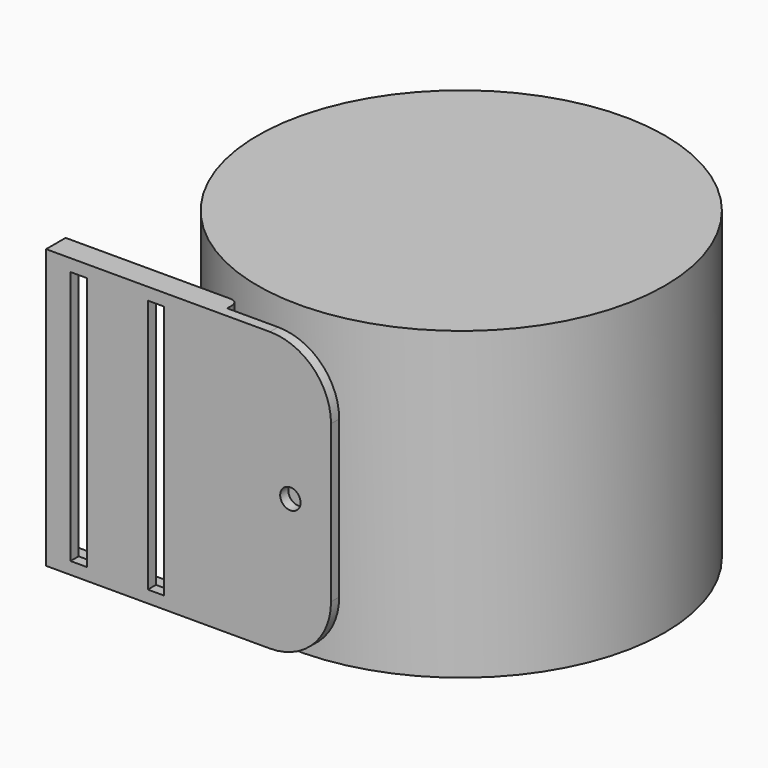
from build123d import *

# Parameters (mm, degrees)
F0_W        = 140
F0_H        = 137
F0_R        = 5
F0_W_2      = 8
F0_H_2      = 125
F1_DEPTH    = 5
F2_R        = 30
F3_R        = 30
F4_W        = 85
F4_H        = 7
F5_DEPTH    = 5
F6_T1_DEPTH = 132.5735082217
F7_W        = 85
F7_H        = 5
F8_DEPTH    = 7
F9_R        = 4
F10_R       = 100.0006041304
F11_DEPTH   = 150


# Not quite as in the source:
# - a fillet or chamfer that OpenCascade refuses, or shapes differently, is made with other operations: its cross-section is extruded or revolved along the edge and cut away or added


with BuildPart() as f1:
    # F0 (on Front) → F1 (new body)
    with BuildSketch(Plane.XZ):
        with Locations((-70, 68.5)):
            Rectangle(F0_W, F0_H)
        Polygon((-128, 5.9977934385), (-128, 130.9977934385), (-120, 130.9977934385), (-120, 6), (-120, 5.9977934385), align=None, mode=Mode.SUBTRACT)
        with Locations((-19.9747101513, 67.9977461696)):
            Circle(F0_R, mode=Mode.SUBTRACT)
        with Locations((-86, 68.5)):
            Rectangle(F0_W_2, F0_H_2, mode=Mode.SUBTRACT)
    extrude(amount=F1_DEPTH)

    # F2
    f2_edges = [f1.edges().sort_by_distance(p)[0] for p in [
        (0, -2.5, 137),
    ]]
    fillet(f2_edges, radius=F2_R)

    # F3
    f3_edges = [f1.edges().sort_by_distance(p)[0] for p in [
        (0, -2.5, 0),
    ]]
    fillet(f3_edges, radius=F3_R)

    # F4 (on Top) → F5 (join)
    with BuildSketch(Plane.XY):
        with Locations((-97.5, 3.5)):
            Rectangle(F4_W, F4_H)
    extrude(amount=F5_DEPTH)

    # F6: fillet of radius 50 on 1 edges, made by hand

    # F6_s2 → F6_t1 (cut)
    with BuildSketch(Plane.XY.offset(-63.7867541109)):
        with BuildLine():
            ThreePointArc((-80.5147016443, 7), (-67.285945089, 5.218253805), (-55, 0))
            Line((-55, 0), (-55, 7))
            Line((-55, 7), (-80.5147016443, 7))
        make_face()
    extrude(amount=F6_T1_DEPTH, mode=Mode.SUBTRACT)

    # F7 (on Front) → F8 (join)
    with BuildSketch(Plane.XZ):
        with Locations((-97.5, 134.5)):
            Rectangle(F7_W, F7_H)
    extrude(amount=-F8_DEPTH)

    # F9
    f9_edges = [f1.edges().sort_by_distance(p)[0] for p in [
        (-55, 7, 134.5),
    ]]
    fillet(f9_edges, radius=F9_R)


with BuildPart() as f11:
    # F10 (on Top) → F11 (new body)
    with BuildSketch(Plane.XY):
        with Locations((-19.999999553, 100.0006041304)):
            Circle(F10_R)
    extrude(amount=F11_DEPTH)


solid = Compound([f1.part, f11.part])
